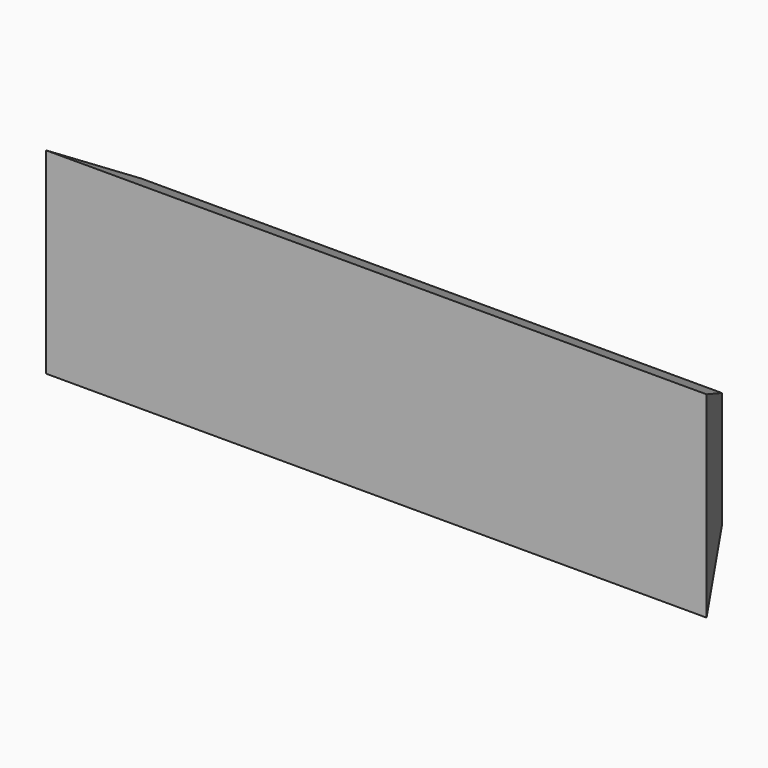
from build123d import *

# Parameters (mm, degrees)
F0_W     = 213.2476568222
F0_H     = 42.8796173073
F1_DEPTH = 25.4
F1_TAPER = -30


# Not quite as in the source:
# - a feature of the source that left no trace in its solid (it failed there, or was rolled back) is left out


with BuildPart() as f1:
    # F0 (on Front) → F1 (new body)
    with BuildSketch(Plane.XZ):
        with Locations((14.4204348326, 14.6504088771)):
            Rectangle(F0_W, F0_H)
    extrude(amount=F1_DEPTH, taper=F1_TAPER)


solid = f1.part
